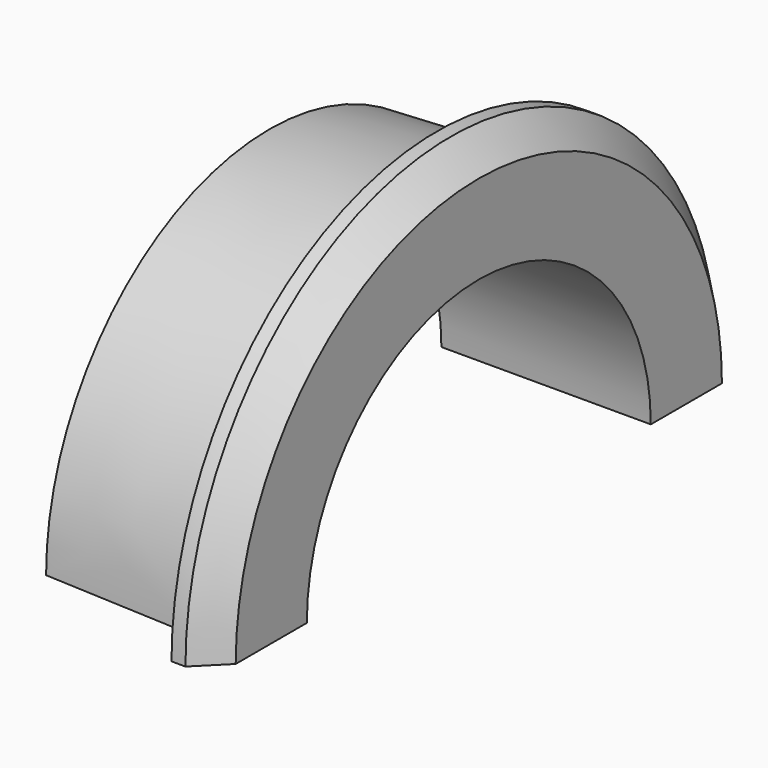
from build123d import *

# Parameters (mm, degrees)
F2_ANGLE_BACK = 90
F2_ANGLE      = 180
F3_SIZE       = 2.54


with BuildPart() as f2:
    # F0 (on Front) → F2 (revolve)
    with BuildSketch(Plane.XZ, mode=Mode.PRIVATE) as f2_sk:
        Polygon((2.9366673195, 26.162), (-12.3033326805, 25.4), (-12.3033326805, 19.558), (6.7466673195, 19.558), (6.7466673195, 30.1889932623), (2.9366673195, 30.1889932623), align=None)
    revolve(f2_sk.sketch.rotate(Axis((-24.6385950595, 0, 0), (-1, 0, 0)), -F2_ANGLE_BACK), axis=Axis((-24.6385950595, 0, 0), (-1, 0, 0)), revolution_arc=F2_ANGLE)

    # F3
    f3_edges = [f2.edges().sort_by_distance(p)[0] for p in [
        (6.746667, 0, 30.188993),
    ]]
    chamfer(f3_edges, length=F3_SIZE)


solid = f2.part
